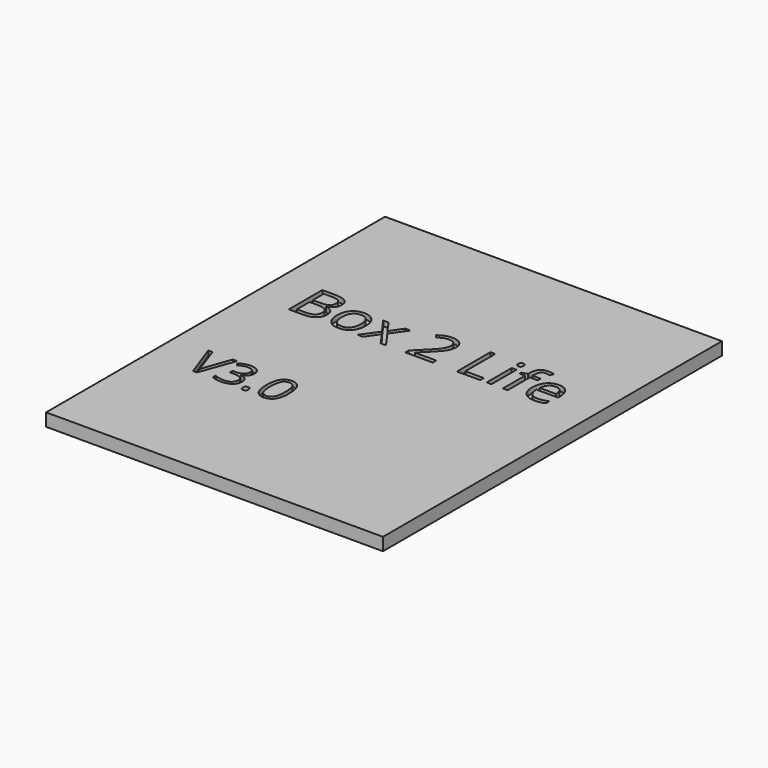
from build123d import *

# Parameters (mm, degrees)
F0_W           = 66
F0_H           = 83
F1_DEPTH       = 2.5
F2_TEXT_SIZE   = 11.4856856979
F2_TEXT_SIZE_2 = 9.5053963984
F3_DEPTH       = 1


# Not quite as in the source:
# - Text() gives the source's letters only with a copy of the font that has no kerning and outlines rounded to 1/6400 em; it was checked with that copy


with BuildPart() as f1:
    # F0 (on Top) → F1 (new body)
    with BuildSketch(Plane.XY):
        with Locations((33, 41.5)):
            Rectangle(F0_W, F0_H)
    extrude(amount=F1_DEPTH)

    # F2 (on face) → F3 (cut)
    with BuildSketch(Plane.XY.offset(2.5)):
        with Locations((6.5587246791, 49.8330034316)):
            Text('Box 2 Life', F2_TEXT_SIZE, font='Open Sans', text_align=(TextAlign.LEFT, TextAlign.BOTTOM))
        with Locations((6.5587246791, 24.7387569398)):
            Text('V3.0', F2_TEXT_SIZE_2, font='Open Sans', text_align=(TextAlign.LEFT, TextAlign.BOTTOM))
    extrude(amount=-F3_DEPTH, mode=Mode.SUBTRACT)


solid = f1.part
